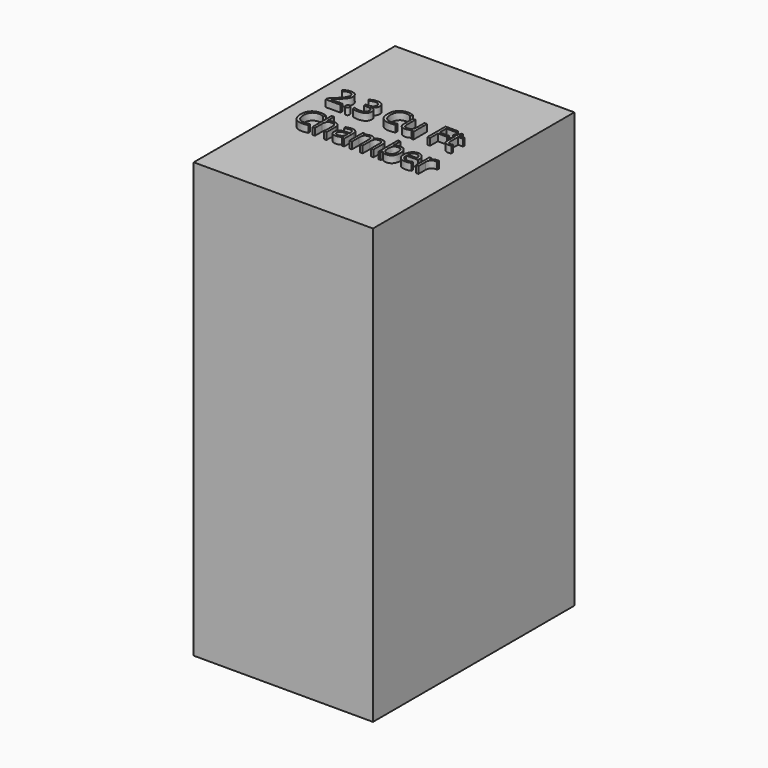
from build123d import *

# Parameters (mm, degrees)
F0_W         = 660.4
F0_H         = 927.1
F1_DEPTH     = 1600.2
F2_TEXT_SIZE = 116.4136350616
F3_DEPTH     = 25.4


# Not quite as in the source:
# - Text() gives the source's letters only with a copy of the font that has no kerning and outlines rounded to 1/6400 em; it was checked with that copy


with BuildPart() as f1:
    # F0 (on Top) → F1 (new body)
    with BuildSketch(Plane.XY):
        Rectangle(F0_W, F0_H)
    extrude(amount=F1_DEPTH)

    # F2 (on face) → F3 (join)
    with BuildSketch(Plane.XY.offset(1600.2)):
        with Locations((-254, 41.6760821507)):
            Text('2.3 Cu Ft', F2_TEXT_SIZE, font='Open Sans', text_align=(TextAlign.LEFT, TextAlign.BOTTOM))
        with Locations((-254, -116.6464615331)):
            Text('Chamber', F2_TEXT_SIZE, font='Open Sans', text_align=(TextAlign.LEFT, TextAlign.BOTTOM))
    extrude(amount=F3_DEPTH)


solid = f1.part
